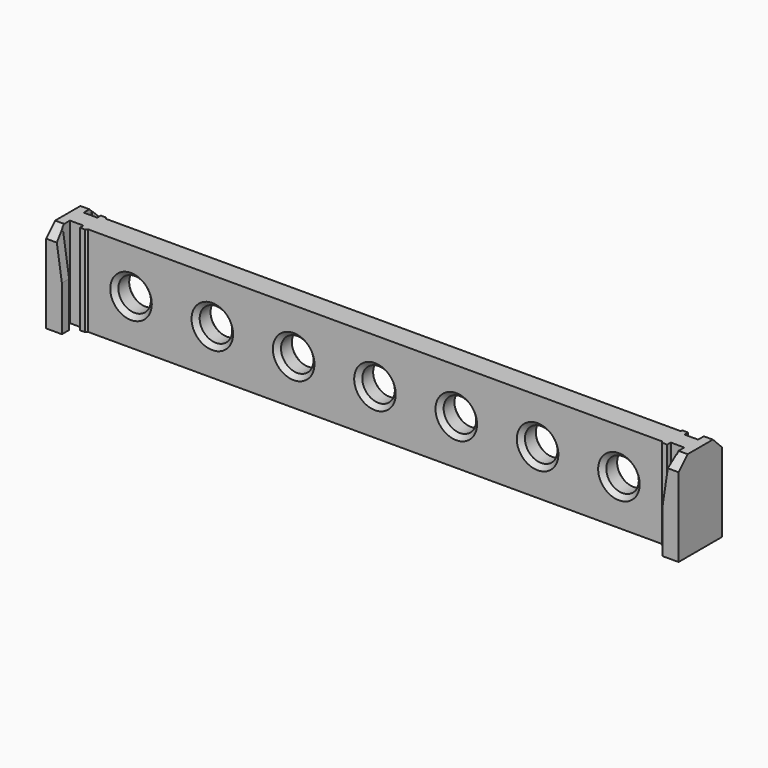
from build123d import *

# Parameters (mm, degrees)
F1_DEPTH     = 20
F2_T4_DEPTH  = 20
F2_T9_DEPTH  = 20
F2_T14_DEPTH = 20
F2_T19_DEPTH = 20
F3_SIZE2     = 1.5
F3_SIZE      = 10
F3_2_SIZE2   = 1.5
F3_2_SIZE    = 10
F3_3_SIZE2   = 1.5
F3_3_SIZE    = 10
F3_4_SIZE2   = 1.5
F3_4_SIZE    = 10
F4_T1_DEPTH  = 14.8584149398
F4_T3_DEPTH  = 14.8584149398
F5_R         = 3.6
F6_DEPTH     = 25
F7_SIZE      = 1


# Not quite as in the source:
# - a fillet or chamfer that OpenCascade refuses, or shapes differently, is made with other operations: its cross-section is extruded or revolved along the edge and cut away or added


with BuildPart() as f1:
    # F0 (on Top) → F1 (new body)
    with BuildSketch(Plane.XY):
        Polygon((-70, 6), (-70, 0), (-70, -6), (-66.5, -6), (-66.5, -4), (-68, -4), (-68, -1.9), (-65, -1.9), (-65, -2.9), (-64, -2.9), (-64, -2.5), (0, -2.5), (64, -2.5), (64, -2.9), (65, -2.9), (65, -1.9), (68, -1.9), (68, -4), (66.5, -4), (66.5, -6), (70, -6), (70, 0), (70, 6), (66.5, 6), (66.5, 4), (68, 4), (68, 1.9), (65, 1.9), (65, 2.9), (64, 2.9), (64, 2.5), (0, 2.5), (-64, 2.5), (-64, 2.9), (-65, 2.9), (-65, 1.9), (-68, 1.9), (-68, 4), (-66.5, 4), (-66.5, 6), align=None)
    extrude(amount=F1_DEPTH)

    # F2: chamfer of 0.5 on 4 edges, made by hand


with BuildPart() as f2_tool2:
    # F2_s3 → F2_t4 (new body)
    with BuildSketch(Plane.XY):
        Polygon((-64, 3), (-63.5, 2.5), (-64, 2.5), align=None)
    extrude(amount=F2_T4_DEPTH)

    split(bisect_by=Plane.XZ.offset(-2.9), keep=Keep.TOP)


with BuildPart() as f1_1:
    add(f1.part)

    # F2_t1: union F2_tool2
    add(f2_tool2.part)


with BuildPart() as f2_tool7:
    # F2_s8 → F2_t9 (new body)
    with BuildSketch(Plane.XY):
        Polygon((-63.5, -2.5), (-64, -3), (-64, -2.5), align=None)
    extrude(amount=F2_T9_DEPTH)

    split(bisect_by=Plane.XZ.offset(2.9), keep=Keep.BOTTOM)


with BuildPart() as f1_2:
    add(f1_1.part)

    # F2_t6: union F2_tool7
    add(f2_tool7.part)


with BuildPart() as f2_tool12:
    # F2_s13 → F2_t14 (new body)
    with BuildSketch(Plane.XY):
        Polygon((64, -3), (63.5, -2.5), (64, -2.5), align=None)
    extrude(amount=F2_T14_DEPTH)

    split(bisect_by=Plane.XZ.offset(2.9), keep=Keep.BOTTOM)


with BuildPart() as f1_3:
    add(f1_2.part)

    # F2_t11: union F2_tool12
    add(f2_tool12.part)


with BuildPart() as f2_tool17:
    # F2_s18 → F2_t19 (new body)
    with BuildSketch(Plane.XY):
        Polygon((63.5, 2.5), (64, 3), (64, 2.5), align=None)
    extrude(amount=F2_T19_DEPTH)

    split(bisect_by=Plane.XZ.offset(-2.9), keep=Keep.TOP)


with BuildPart() as f1_4:
    add(f1_3.part)

    # F2_t16: union F2_tool17
    add(f2_tool17.part)

    # F3
    f3_edges = [f1_4.edges().sort_by_distance(p)[0] for p in [
        (-66.5, 5, 20),
    ]]
    f3_side = f1_4.faces().sort_by_distance((-66.5, 5, 10))[0]
    chamfer(f3_edges, length=F3_SIZE, length2=F3_SIZE2, reference=f3_side)

    # F3#2
    f3_2_edges = [f1_4.edges().sort_by_distance(p)[0] for p in [
        (-66.5, -5, 20),
    ]]
    f3_2_side = f1_4.faces().sort_by_distance((-66.5, -5, 10))[0]
    chamfer(f3_2_edges, length=F3_2_SIZE, length2=F3_2_SIZE2, reference=f3_2_side)

    # F3#3
    f3_3_edges = [f1_4.edges().sort_by_distance(p)[0] for p in [
        (66.5, 5, 20),
    ]]
    f3_3_side = f1_4.faces().sort_by_distance((66.5, 5, 10))[0]
    chamfer(f3_3_edges, length=F3_3_SIZE, length2=F3_3_SIZE2, reference=f3_3_side)

    # F3#4
    f3_4_edges = [f1_4.edges().sort_by_distance(p)[0] for p in [
        (66.5, -5, 20),
    ]]
    f3_4_side = f1_4.faces().sort_by_distance((66.5, -5, 10))[0]
    chamfer(f3_4_edges, length=F3_4_SIZE, length2=F3_4_SIZE2, reference=f3_4_side)

    # F4: chamfer of 2.5 on 4 edges, made by hand

    # F4_s2 → F4_t1 (cut)
    with BuildSketch(Plane.YZ.offset(-76.4292074699)):
        Polygon((3.5, 20), (6, 17.5), (6, 20), align=None)
        Polygon((-3.5, 20), (-6, 17.5), (-6, 20), align=None)
    extrude(amount=F4_T1_DEPTH, mode=Mode.SUBTRACT)

    # F4_s4 → F4_t3 (cut)
    with BuildSketch(Plane.YZ.offset(61.5707925301)):
        Polygon((3.5, 20), (6, 17.5), (6, 20), align=None)
        Polygon((-3.5, 20), (-6, 17.5), (-6, 20), align=None)
    extrude(amount=F4_T3_DEPTH, mode=Mode.SUBTRACT)

    # F5 (on face) → F6 (cut)
    with BuildSketch(Plane.XZ.offset(2.5)):
        with Locations((-54, 10)):
            Circle(F5_R)
        with Locations((-36, 10)):
            Circle(F5_R)
        with Locations((-18, 10)):
            Circle(F5_R)
        with Locations((0, 10)):
            Circle(F5_R)
        with Locations((18, 10)):
            Circle(F5_R)
        with Locations((36, 10)):
            Circle(F5_R)
        with Locations((54, 10)):
            Circle(F5_R)
    extrude(amount=-F6_DEPTH, mode=Mode.SUBTRACT)

    # F7
    f7_edges = [f1_4.edges().sort_by_distance(p)[0] for p in [
        (-57.6, -2.5, 10),
        (-50.4, 0, 10),
        (-57.6, 2.5, 10),
        (-39.6, -2.5, 10),
        (-32.4, 0, 10),
        (-39.6, 2.5, 10),
        (-21.6, -2.5, 10),
        (-14.4, 0, 10),
        (-21.6, 2.5, 10),
        (-3.6, -2.5, 10),
        (3.6, 0, 10),
        (-3.6, 2.5, 10),
        (14.4, -2.5, 10),
        (21.6, 0, 10),
        (14.4, 2.5, 10),
        (32.4, -2.5, 10),
        (39.6, 0, 10),
        (32.4, 2.5, 10),
        (50.4, -2.5, 10),
        (57.6, 0, 10),
        (50.4, 2.5, 10),
    ]]
    chamfer(f7_edges, length=F7_SIZE)


solid = f1_4.part
